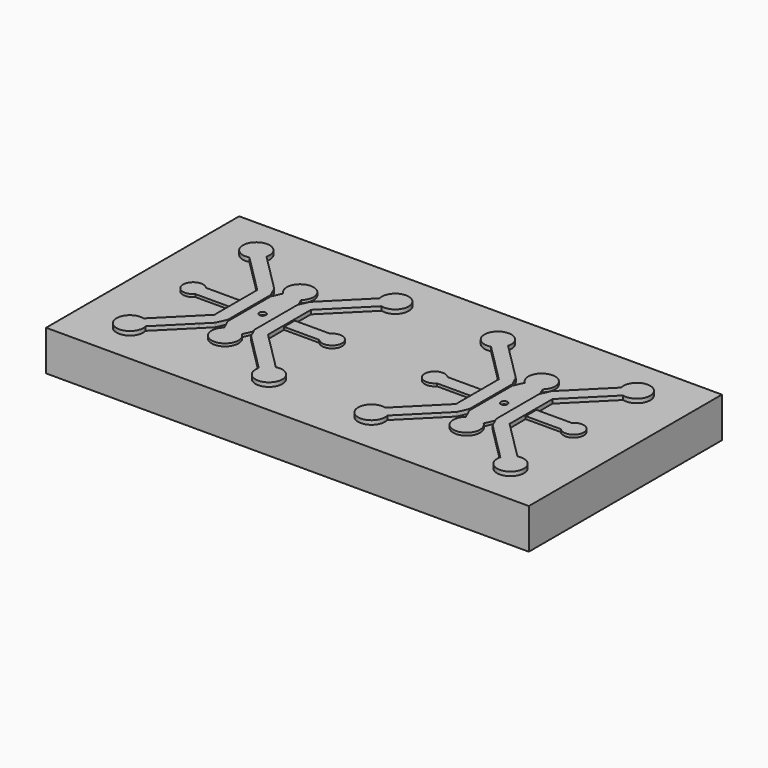
from build123d import *

# Parameters (mm, degrees)
F0_W     = 17.75
F0_H     = 18
F0_W_2   = 0.25
F1_DEPTH = 3
F2_DEPTH = 0.3
F3_DEPTH = 0.2


# Not quite as in the source:
# - a feature names something its author has since deleted; it is built from what else it names


with BuildPart() as f1:
    # F0 (on Top) → F1 (new body)
    with BuildSketch(Plane.XY):
        with Locations((8.875, 9)):
            Rectangle(F0_W, F0_H)
        with BuildLine():
            Line((9.6533412223, 11.6952957055), (9.9919033945, 10.9452957055))
            Line((9.9919033945, 10.9452957055), (10.3304655668, 11.6952957055))
            Line((10.3304655668, 11.6952957055), (10.9904227081, 12.3580254744))
            Line((10.9904227081, 12.3580254744), (13.2079580316, 14.5755632326))
            ThreePointArc((13.2079580316, 14.5755632326), (14.8809903029, 15.5414897832), (13.9150646707, 13.8684569817))
            Line((13.9150646707, 13.8684569817), (10.9919033945, 10.9452957055))
            Line((10.9919033945, 10.9452957055), (10.9919033945, 9.4452957055))
            Line((10.9919033945, 9.4452957055), (13.6148667214, 9.4452957055))
            ThreePointArc((13.6148667214, 9.4452957055), (13.70376764, 9.5296679116), (13.8052234095, 9.5984339593))
            ThreePointArc((13.8052234095, 9.5984339593), (14.9138690208, 8.823141097), (13.6148667214, 8.4452957055))
            Line((13.6148667214, 8.4452957055), (10.9919033945, 8.4452957055))
            Line((10.9919033945, 8.4452957055), (10.9919033945, 6.9452957055))
            Line((10.9919033945, 6.9452957055), (13.9150646707, 4.0221344294))
            ThreePointArc((13.9150646707, 4.0221344294), (14.8809903029, 2.3491016278), (13.2079580316, 3.3150281785))
            Line((13.2079580316, 3.3150281785), (10.9904227081, 5.5325659367))
            Line((10.9904227081, 5.5325659367), (10.3304655668, 6.1952957055))
            Line((10.3304655668, 6.1952957055), (9.9919033945, 6.9452957055))
            Line((9.9919033945, 6.9452957055), (9.6533412223, 6.1952957055))
            ThreePointArc((9.6533412223, 6.1952957055), (8.9919033945, 4.4452957055), (8.3304655668, 6.1952957055))
            Line((8.3304655668, 6.1952957055), (7.9919033945, 6.9452957055))
            Line((7.9919033945, 6.9452957055), (7.6533412223, 6.1952957055))
            Line((7.6533412223, 6.1952957055), (6.993384081, 5.5325659367))
            Line((6.993384081, 5.5325659367), (4.7758487575, 3.3150281785))
            ThreePointArc((4.7758487575, 3.3150281785), (3.1028164862, 2.3491016278), (4.0687421184, 4.0221344294))
            Line((4.0687421184, 4.0221344294), (6.9919033945, 6.9452957055))
            Line((6.9919033945, 6.9452957055), (6.9919033945, 8.4452957055))
            Line((6.9919033945, 8.4452957055), (4.3689400677, 8.4452957055))
            ThreePointArc((4.3689400677, 8.4452957055), (3.0699377683, 8.823141097), (4.1785833795, 9.5984339593))
            ThreePointArc((4.1785833795, 9.5984339593), (4.2800391491, 9.5296679116), (4.3689400677, 9.4452957055))
            Line((4.3689400677, 9.4452957055), (6.9919033945, 9.4452957055))
            Line((6.9919033945, 9.4452957055), (6.9919033945, 10.9452957055))
            Line((6.9919033945, 10.9452957055), (4.0687421184, 13.8684569817))
            ThreePointArc((4.0687421184, 13.8684569817), (3.1028164862, 15.5414897832), (4.7758487575, 14.5755632326))
            Line((4.7758487575, 14.5755632326), (6.993384081, 12.3580254744))
            Line((6.993384081, 12.3580254744), (7.6533412223, 11.6952957055))
            Line((7.6533412223, 11.6952957055), (7.9919033945, 10.9452957055))
            Line((7.9919033945, 10.9452957055), (8.3304655668, 11.6952957055))
            ThreePointArc((8.3304655668, 11.6952957055), (8.9919033945, 13.4452957055), (9.6533412223, 11.6952957055))
        make_face(mode=Mode.SUBTRACT)
        with Locations((27.125, 9)):
            Rectangle(F0_W, F0_H)
        with BuildLine():
            Line((27.6695344332, 11.6952957055), (28.0080966055, 10.9452957055))
            Line((28.0080966055, 10.9452957055), (28.3466587777, 11.6952957055))
            Line((28.3466587777, 11.6952957055), (29.006615919, 12.3580254744))
            Line((29.006615919, 12.3580254744), (31.2241512425, 14.5755632326))
            ThreePointArc((31.2241512425, 14.5755632326), (32.8971835138, 15.5414897832), (31.9312578816, 13.8684569817))
            Line((31.9312578816, 13.8684569817), (29.0080966055, 10.9452957055))
            Line((29.0080966055, 10.9452957055), (29.0080966055, 9.4452957055))
            Line((29.0080966055, 9.4452957055), (31.6310599323, 9.4452957055))
            ThreePointArc((31.6310599323, 9.4452957055), (31.7199608509, 9.5296679116), (31.8214166205, 9.5984339593))
            ThreePointArc((31.8214166205, 9.5984339593), (32.9300622317, 8.823141097), (31.6310599323, 8.4452957055))
            Line((31.6310599323, 8.4452957055), (29.0080966055, 8.4452957055))
            Line((29.0080966055, 8.4452957055), (29.0080966055, 6.9452957055))
            Line((29.0080966055, 6.9452957055), (31.9312578816, 4.0221344294))
            ThreePointArc((31.9312578816, 4.0221344294), (32.8971835138, 2.3491016278), (31.2241512425, 3.3150281785))
            Line((31.2241512425, 3.3150281785), (29.006615919, 5.5325659367))
            Line((29.006615919, 5.5325659367), (28.3466587777, 6.1952957055))
            Line((28.3466587777, 6.1952957055), (28.0080966055, 6.9452957055))
            Line((28.0080966055, 6.9452957055), (27.6695344332, 6.1952957055))
            ThreePointArc((27.6695344332, 6.1952957055), (27.0080966055, 4.4452957055), (26.3466587777, 6.1952957055))
            Line((26.3466587777, 6.1952957055), (26.0080966055, 6.9452957055))
            Line((26.0080966055, 6.9452957055), (25.6695344332, 6.1952957055))
            Line((25.6695344332, 6.1952957055), (25.0095772919, 5.5325659367))
            Line((25.0095772919, 5.5325659367), (22.7920419684, 3.3150281785))
            ThreePointArc((22.7920419684, 3.3150281785), (21.1190096971, 2.3491016278), (22.0849353293, 4.0221344294))
            Line((22.0849353293, 4.0221344294), (25.0080966055, 6.9452957055))
            Line((25.0080966055, 6.9452957055), (25.0080966055, 8.4452957055))
            Line((25.0080966055, 8.4452957055), (22.3851332786, 8.4452957055))
            ThreePointArc((22.3851332786, 8.4452957055), (21.0861309792, 8.823141097), (22.1947765905, 9.5984339593))
            ThreePointArc((22.1947765905, 9.5984339593), (22.29623236, 9.5296679116), (22.3851332786, 9.4452957055))
            Line((22.3851332786, 9.4452957055), (25.0080966055, 9.4452957055))
            Line((25.0080966055, 9.4452957055), (25.0080966055, 10.9452957055))
            Line((25.0080966055, 10.9452957055), (22.0849353293, 13.8684569817))
            ThreePointArc((22.0849353293, 13.8684569817), (21.1190096971, 15.5414897832), (22.7920419684, 14.5755632326))
            Line((22.7920419684, 14.5755632326), (25.0095772919, 12.3580254744))
            Line((25.0095772919, 12.3580254744), (25.6695344332, 11.6952957055))
            Line((25.6695344332, 11.6952957055), (26.0080966055, 10.9452957055))
            Line((26.0080966055, 10.9452957055), (26.3466587777, 11.6952957055))
            ThreePointArc((26.3466587777, 11.6952957055), (27.0080966055, 13.4452957055), (27.6695344332, 11.6952957055))
        make_face(mode=Mode.SUBTRACT)
        with BuildLine():
            Line((26.0080966055, 8.9452957055), (26.0080966055, 10.9452957055))
            Line((26.0080966055, 10.9452957055), (25.6695344332, 11.6952957055))
            Line((25.6695344332, 11.6952957055), (25.0095772919, 12.3580254744))
            Line((25.0095772919, 12.3580254744), (22.7920419684, 14.5755632326))
            ThreePointArc((22.7920419684, 14.5755632326), (21.1190096971, 15.5414897832), (22.0849353293, 13.8684569817))
            Line((22.0849353293, 13.8684569817), (25.0080966055, 10.9452957055))
            Line((25.0080966055, 10.9452957055), (25.0080966055, 9.4452957055))
            Line((25.0080966055, 9.4452957055), (25.0080966055, 8.9452957055))
            Line((25.0080966055, 8.9452957055), (25.0080966055, 8.4452957055))
            Line((25.0080966055, 8.4452957055), (25.0080966055, 6.9452957055))
            Line((25.0080966055, 6.9452957055), (22.0849353293, 4.0221344294))
            ThreePointArc((22.0849353293, 4.0221344294), (21.1190096971, 2.3491016278), (22.7920419684, 3.3150281785))
            Line((22.7920419684, 3.3150281785), (25.0095772919, 5.5325659367))
            Line((25.0095772919, 5.5325659367), (25.6695344332, 6.1952957055))
            Line((25.6695344332, 6.1952957055), (26.0080966055, 6.9452957055))
            Line((26.0080966055, 6.9452957055), (26.0080966055, 8.9452957055))
        make_face()
        with BuildLine():
            Line((28.3466587777, 11.6952957055), (28.0080966055, 10.9452957055))
            Line((28.0080966055, 10.9452957055), (28.0080966055, 8.9452957055))
            Line((28.0080966055, 8.9452957055), (28.0080966055, 6.9452957055))
            Line((28.0080966055, 6.9452957055), (28.3466587777, 6.1952957055))
            Line((28.3466587777, 6.1952957055), (29.006615919, 5.5325659367))
            Line((29.006615919, 5.5325659367), (31.2241512425, 3.3150281785))
            ThreePointArc((31.2241512425, 3.3150281785), (32.8971835138, 2.3491016278), (31.9312578816, 4.0221344294))
            Line((31.9312578816, 4.0221344294), (29.0080966055, 6.9452957055))
            Line((29.0080966055, 6.9452957055), (29.0080966055, 8.4452957055))
            Line((29.0080966055, 8.4452957055), (29.0080966055, 8.9452957055))
            Line((29.0080966055, 8.9452957055), (29.0080966055, 9.4452957055))
            Line((29.0080966055, 9.4452957055), (29.0080966055, 10.9452957055))
            Line((29.0080966055, 10.9452957055), (31.9312578816, 13.8684569817))
            ThreePointArc((31.9312578816, 13.8684569817), (32.8971835138, 15.5414897832), (31.2241512425, 14.5755632326))
            Line((31.2241512425, 14.5755632326), (29.006615919, 12.3580254744))
            Line((29.006615919, 12.3580254744), (28.3466587777, 11.6952957055))
        make_face()
        with BuildLine():
            Line((7.9919033945, 8.9452957055), (7.9919033945, 10.9452957055))
            Line((7.9919033945, 10.9452957055), (7.6533412223, 11.6952957055))
            Line((7.6533412223, 11.6952957055), (6.993384081, 12.3580254744))
            Line((6.993384081, 12.3580254744), (4.7758487575, 14.5755632326))
            ThreePointArc((4.7758487575, 14.5755632326), (3.1028164862, 15.5414897832), (4.0687421184, 13.8684569817))
            Line((4.0687421184, 13.8684569817), (6.9919033945, 10.9452957055))
            Line((6.9919033945, 10.9452957055), (6.9919033945, 9.4452957055))
            Line((6.9919033945, 9.4452957055), (6.9919033945, 8.9452957055))
            Line((6.9919033945, 8.9452957055), (6.9919033945, 8.4452957055))
            Line((6.9919033945, 8.4452957055), (6.9919033945, 6.9452957055))
            Line((6.9919033945, 6.9452957055), (4.0687421184, 4.0221344294))
            ThreePointArc((4.0687421184, 4.0221344294), (3.1028164862, 2.3491016278), (4.7758487575, 3.3150281785))
            Line((4.7758487575, 3.3150281785), (6.993384081, 5.5325659367))
            Line((6.993384081, 5.5325659367), (7.6533412223, 6.1952957055))
            Line((7.6533412223, 6.1952957055), (7.9919033945, 6.9452957055))
            Line((7.9919033945, 6.9452957055), (7.9919033945, 8.9452957055))
        make_face()
        with BuildLine():
            Line((9.9919033945, 10.9452957055), (9.9919033945, 8.9452957055))
            Line((9.9919033945, 8.9452957055), (9.9919033945, 6.9452957055))
            Line((9.9919033945, 6.9452957055), (10.3304655668, 6.1952957055))
            Line((10.3304655668, 6.1952957055), (10.9904227081, 5.5325659367))
            Line((10.9904227081, 5.5325659367), (13.2079580316, 3.3150281785))
            ThreePointArc((13.2079580316, 3.3150281785), (14.8809903029, 2.3491016278), (13.9150646707, 4.0221344294))
            Line((13.9150646707, 4.0221344294), (10.9919033945, 6.9452957055))
            Line((10.9919033945, 6.9452957055), (10.9919033945, 8.4452957055))
            Line((10.9919033945, 8.4452957055), (10.9919033945, 8.9452957055))
            Line((10.9919033945, 8.9452957055), (10.9919033945, 9.4452957055))
            Line((10.9919033945, 9.4452957055), (10.9919033945, 10.9452957055))
            Line((10.9919033945, 10.9452957055), (13.9150646707, 13.8684569817))
            ThreePointArc((13.9150646707, 13.8684569817), (14.8809903029, 15.5414897832), (13.2079580316, 14.5755632326))
            Line((13.2079580316, 14.5755632326), (10.9904227081, 12.3580254744))
            Line((10.9904227081, 12.3580254744), (10.3304655668, 11.6952957055))
            Line((10.3304655668, 11.6952957055), (9.9919033945, 10.9452957055))
        make_face()
        with BuildLine():
            Line((28.0080966055, 8.9452957055), (28.0080966055, 10.9452957055))
            Line((28.0080966055, 10.9452957055), (27.6695344332, 11.6952957055))
            ThreePointArc((27.6695344332, 11.6952957055), (27.0080966055, 13.4452957055), (26.3466587777, 11.6952957055))
            Line((26.3466587777, 11.6952957055), (26.0080966055, 10.9452957055))
            Line((26.0080966055, 10.9452957055), (26.0080966055, 8.9452957055))
            Line((26.0080966055, 8.9452957055), (26.0080966055, 6.9452957055))
            Line((26.0080966055, 6.9452957055), (26.3466587777, 6.1952957055))
            ThreePointArc((26.3466587777, 6.1952957055), (27.0080966055, 4.4452957055), (27.6695344332, 6.1952957055))
            Line((27.6695344332, 6.1952957055), (28.0080966055, 6.9452957055))
            Line((28.0080966055, 6.9452957055), (28.0080966055, 8.9452957055))
        make_face()
        with BuildLine():
            ThreePointArc((27.0080966055, 9.1952957055), (27.1848733008, 9.1220724008), (27.2580966055, 8.9452957055))
            ThreePointArc((27.2580966055, 8.9452957055), (27.1848733008, 8.7685190102), (27.0080966055, 8.6952957055))
            ThreePointArc((27.0080966055, 8.6952957055), (26.7580966055, 8.9452957055), (27.0080966055, 9.1952957055))
        make_face(mode=Mode.SUBTRACT)
        with BuildLine():
            Line((9.9919033945, 6.9452957055), (9.9919033945, 8.9452957055))
            Line((9.9919033945, 8.9452957055), (9.9919033945, 10.9452957055))
            Line((9.9919033945, 10.9452957055), (9.6533412223, 11.6952957055))
            ThreePointArc((9.6533412223, 11.6952957055), (8.9919033945, 13.4452957055), (8.3304655668, 11.6952957055))
            Line((8.3304655668, 11.6952957055), (7.9919033945, 10.9452957055))
            Line((7.9919033945, 10.9452957055), (7.9919033945, 8.9452957055))
            Line((7.9919033945, 8.9452957055), (7.9919033945, 6.9452957055))
            Line((7.9919033945, 6.9452957055), (8.3304655668, 6.1952957055))
            ThreePointArc((8.3304655668, 6.1952957055), (8.9919033945, 4.4452957055), (9.6533412223, 6.1952957055))
            Line((9.6533412223, 6.1952957055), (9.9919033945, 6.9452957055))
        make_face()
        with BuildLine():
            ThreePointArc((8.9919033945, 9.1952957055), (9.1686800898, 9.1220724008), (9.2419033945, 8.9452957055))
            ThreePointArc((9.2419033945, 8.9452957055), (9.1686800898, 8.7685190102), (8.9919033945, 8.6952957055))
            ThreePointArc((8.9919033945, 8.6952957055), (8.7419033945, 8.9452957055), (8.9919033945, 9.1952957055))
        make_face(mode=Mode.SUBTRACT)
        with Locations((17.875, 9)):
            Rectangle(F0_W_2, F0_H)
        with Locations((18.125, 9)):
            Rectangle(F0_W_2, F0_H)
        with BuildLine():
            Line((6.9919033945, 8.9452957055), (6.9919033945, 9.4452957055))
            Line((6.9919033945, 9.4452957055), (4.3689400677, 9.4452957055))
            ThreePointArc((4.3689400677, 9.4452957055), (4.2800391491, 9.5296679116), (4.1785833795, 9.5984339593))
            ThreePointArc((4.1785833795, 9.5984339593), (3.0699377683, 8.823141097), (4.3689400677, 8.4452957055))
            Line((4.3689400677, 8.4452957055), (6.9919033945, 8.4452957055))
            Line((6.9919033945, 8.4452957055), (6.9919033945, 8.9452957055))
        make_face()
        with BuildLine():
            Line((31.6310599323, 9.4452957055), (29.0080966055, 9.4452957055))
            Line((29.0080966055, 9.4452957055), (29.0080966055, 8.9452957055))
            Line((29.0080966055, 8.9452957055), (29.0080966055, 8.4452957055))
            Line((29.0080966055, 8.4452957055), (31.6310599323, 8.4452957055))
            ThreePointArc((31.6310599323, 8.4452957055), (32.9300622317, 8.823141097), (31.8214166205, 9.5984339593))
            ThreePointArc((31.8214166205, 9.5984339593), (31.7199608509, 9.5296679116), (31.6310599323, 9.4452957055))
        make_face()
        with BuildLine():
            Line((25.0080966055, 8.9452957055), (25.0080966055, 9.4452957055))
            Line((25.0080966055, 9.4452957055), (22.3851332786, 9.4452957055))
            ThreePointArc((22.3851332786, 9.4452957055), (22.29623236, 9.5296679116), (22.1947765905, 9.5984339593))
            ThreePointArc((22.1947765905, 9.5984339593), (21.0861309792, 8.823141097), (22.3851332786, 8.4452957055))
            Line((22.3851332786, 8.4452957055), (25.0080966055, 8.4452957055))
            Line((25.0080966055, 8.4452957055), (25.0080966055, 8.9452957055))
        make_face()
        with BuildLine():
            Line((13.6148667214, 9.4452957055), (10.9919033945, 9.4452957055))
            Line((10.9919033945, 9.4452957055), (10.9919033945, 8.9452957055))
            Line((10.9919033945, 8.9452957055), (10.9919033945, 8.4452957055))
            Line((10.9919033945, 8.4452957055), (13.6148667214, 8.4452957055))
            ThreePointArc((13.6148667214, 8.4452957055), (14.9138690208, 8.823141097), (13.8052234095, 9.5984339593))
            ThreePointArc((13.8052234095, 9.5984339593), (13.70376764, 9.5296679116), (13.6148667214, 9.4452957055))
        make_face()
        with BuildLine():
            ThreePointArc((8.9919033945, 8.6952957055), (9.1686800898, 8.7685190102), (9.2419033945, 8.9452957055))
            ThreePointArc((9.2419033945, 8.9452957055), (9.1686800898, 9.1220724008), (8.9919033945, 9.1952957055))
            Line((8.9919033945, 9.1952957055), (8.9919033945, 8.6952957055))
        make_face()
        with BuildLine():
            ThreePointArc((27.0080966055, 8.6952957055), (27.1848733008, 8.7685190102), (27.2580966055, 8.9452957055))
            ThreePointArc((27.2580966055, 8.9452957055), (27.1848733008, 9.1220724008), (27.0080966055, 9.1952957055))
            Line((27.0080966055, 9.1952957055), (27.0080966055, 8.6952957055))
        make_face()
        with BuildLine():
            Line((8.9919033945, 8.6952957055), (8.9919033945, 9.1952957055))
            ThreePointArc((8.9919033945, 9.1952957055), (8.7419033945, 8.9452957055), (8.9919033945, 8.6952957055))
        make_face()
        with BuildLine():
            Line((27.0080966055, 8.6952957055), (27.0080966055, 9.1952957055))
            ThreePointArc((27.0080966055, 9.1952957055), (26.7580966055, 8.9452957055), (27.0080966055, 8.6952957055))
        make_face()
    extrude(amount=-F1_DEPTH)

    # F0 (on Top) → F2 (join)
    with BuildSketch(Plane.XY):
        with BuildLine():
            Line((7.9919033945, 8.9452957055), (7.9919033945, 10.9452957055))
            Line((7.9919033945, 10.9452957055), (7.6533412223, 11.6952957055))
            Line((7.6533412223, 11.6952957055), (6.993384081, 12.3580254744))
            Line((6.993384081, 12.3580254744), (4.7758487575, 14.5755632326))
            ThreePointArc((4.7758487575, 14.5755632326), (3.1028164862, 15.5414897832), (4.0687421184, 13.8684569817))
            Line((4.0687421184, 13.8684569817), (6.9919033945, 10.9452957055))
            Line((6.9919033945, 10.9452957055), (6.9919033945, 9.4452957055))
            Line((6.9919033945, 9.4452957055), (6.9919033945, 8.9452957055))
            Line((6.9919033945, 8.9452957055), (6.9919033945, 8.4452957055))
            Line((6.9919033945, 8.4452957055), (6.9919033945, 6.9452957055))
            Line((6.9919033945, 6.9452957055), (4.0687421184, 4.0221344294))
            ThreePointArc((4.0687421184, 4.0221344294), (3.1028164862, 2.3491016278), (4.7758487575, 3.3150281785))
            Line((4.7758487575, 3.3150281785), (6.993384081, 5.5325659367))
            Line((6.993384081, 5.5325659367), (7.6533412223, 6.1952957055))
            Line((7.6533412223, 6.1952957055), (7.9919033945, 6.9452957055))
            Line((7.9919033945, 6.9452957055), (7.9919033945, 8.9452957055))
        make_face()
        with BuildLine():
            Line((9.9919033945, 10.9452957055), (9.9919033945, 8.9452957055))
            Line((9.9919033945, 8.9452957055), (9.9919033945, 6.9452957055))
            Line((9.9919033945, 6.9452957055), (10.3304655668, 6.1952957055))
            Line((10.3304655668, 6.1952957055), (10.9904227081, 5.5325659367))
            Line((10.9904227081, 5.5325659367), (13.2079580316, 3.3150281785))
            ThreePointArc((13.2079580316, 3.3150281785), (14.8809903029, 2.3491016278), (13.9150646707, 4.0221344294))
            Line((13.9150646707, 4.0221344294), (10.9919033945, 6.9452957055))
            Line((10.9919033945, 6.9452957055), (10.9919033945, 8.4452957055))
            Line((10.9919033945, 8.4452957055), (10.9919033945, 8.9452957055))
            Line((10.9919033945, 8.9452957055), (10.9919033945, 9.4452957055))
            Line((10.9919033945, 9.4452957055), (10.9919033945, 10.9452957055))
            Line((10.9919033945, 10.9452957055), (13.9150646707, 13.8684569817))
            ThreePointArc((13.9150646707, 13.8684569817), (14.8809903029, 15.5414897832), (13.2079580316, 14.5755632326))
            Line((13.2079580316, 14.5755632326), (10.9904227081, 12.3580254744))
            Line((10.9904227081, 12.3580254744), (10.3304655668, 11.6952957055))
            Line((10.3304655668, 11.6952957055), (9.9919033945, 10.9452957055))
        make_face()
        with BuildLine():
            Line((26.0080966055, 8.9452957055), (26.0080966055, 10.9452957055))
            Line((26.0080966055, 10.9452957055), (25.6695344332, 11.6952957055))
            Line((25.6695344332, 11.6952957055), (25.0095772919, 12.3580254744))
            Line((25.0095772919, 12.3580254744), (22.7920419684, 14.5755632326))
            ThreePointArc((22.7920419684, 14.5755632326), (21.1190096971, 15.5414897832), (22.0849353293, 13.8684569817))
            Line((22.0849353293, 13.8684569817), (25.0080966055, 10.9452957055))
            Line((25.0080966055, 10.9452957055), (25.0080966055, 9.4452957055))
            Line((25.0080966055, 9.4452957055), (25.0080966055, 8.9452957055))
            Line((25.0080966055, 8.9452957055), (25.0080966055, 8.4452957055))
            Line((25.0080966055, 8.4452957055), (25.0080966055, 6.9452957055))
            Line((25.0080966055, 6.9452957055), (22.0849353293, 4.0221344294))
            ThreePointArc((22.0849353293, 4.0221344294), (21.1190096971, 2.3491016278), (22.7920419684, 3.3150281785))
            Line((22.7920419684, 3.3150281785), (25.0095772919, 5.5325659367))
            Line((25.0095772919, 5.5325659367), (25.6695344332, 6.1952957055))
            Line((25.6695344332, 6.1952957055), (26.0080966055, 6.9452957055))
            Line((26.0080966055, 6.9452957055), (26.0080966055, 8.9452957055))
        make_face()
        with BuildLine():
            Line((28.3466587777, 11.6952957055), (28.0080966055, 10.9452957055))
            Line((28.0080966055, 10.9452957055), (28.0080966055, 8.9452957055))
            Line((28.0080966055, 8.9452957055), (28.0080966055, 6.9452957055))
            Line((28.0080966055, 6.9452957055), (28.3466587777, 6.1952957055))
            Line((28.3466587777, 6.1952957055), (29.006615919, 5.5325659367))
            Line((29.006615919, 5.5325659367), (31.2241512425, 3.3150281785))
            ThreePointArc((31.2241512425, 3.3150281785), (32.8971835138, 2.3491016278), (31.9312578816, 4.0221344294))
            Line((31.9312578816, 4.0221344294), (29.0080966055, 6.9452957055))
            Line((29.0080966055, 6.9452957055), (29.0080966055, 8.4452957055))
            Line((29.0080966055, 8.4452957055), (29.0080966055, 8.9452957055))
            Line((29.0080966055, 8.9452957055), (29.0080966055, 9.4452957055))
            Line((29.0080966055, 9.4452957055), (29.0080966055, 10.9452957055))
            Line((29.0080966055, 10.9452957055), (31.9312578816, 13.8684569817))
            ThreePointArc((31.9312578816, 13.8684569817), (32.8971835138, 15.5414897832), (31.2241512425, 14.5755632326))
            Line((31.2241512425, 14.5755632326), (29.006615919, 12.3580254744))
            Line((29.006615919, 12.3580254744), (28.3466587777, 11.6952957055))
        make_face()
    extrude(amount=F2_DEPTH)

    # F0 (on Top) → F3 (join)
    with BuildSketch(Plane.XY):
        with BuildLine():
            Line((9.9919033945, 6.9452957055), (9.9919033945, 8.9452957055))
            Line((9.9919033945, 8.9452957055), (9.9919033945, 10.9452957055))
            Line((9.9919033945, 10.9452957055), (9.6533412223, 11.6952957055))
            ThreePointArc((9.6533412223, 11.6952957055), (8.9919033945, 13.4452957055), (8.3304655668, 11.6952957055))
            Line((8.3304655668, 11.6952957055), (7.9919033945, 10.9452957055))
            Line((7.9919033945, 10.9452957055), (7.9919033945, 8.9452957055))
            Line((7.9919033945, 8.9452957055), (7.9919033945, 6.9452957055))
            Line((7.9919033945, 6.9452957055), (8.3304655668, 6.1952957055))
            ThreePointArc((8.3304655668, 6.1952957055), (8.9919033945, 4.4452957055), (9.6533412223, 6.1952957055))
            Line((9.6533412223, 6.1952957055), (9.9919033945, 6.9452957055))
        make_face()
        with BuildLine():
            ThreePointArc((8.9919033945, 9.1952957055), (9.1686800898, 9.1220724008), (9.2419033945, 8.9452957055))
            ThreePointArc((9.2419033945, 8.9452957055), (9.1686800898, 8.7685190102), (8.9919033945, 8.6952957055))
            ThreePointArc((8.9919033945, 8.6952957055), (8.7419033945, 8.9452957055), (8.9919033945, 9.1952957055))
        make_face(mode=Mode.SUBTRACT)
        with BuildLine():
            Line((13.6148667214, 9.4452957055), (10.9919033945, 9.4452957055))
            Line((10.9919033945, 9.4452957055), (10.9919033945, 8.9452957055))
            Line((10.9919033945, 8.9452957055), (10.9919033945, 8.4452957055))
            Line((10.9919033945, 8.4452957055), (13.6148667214, 8.4452957055))
            ThreePointArc((13.6148667214, 8.4452957055), (14.9138690208, 8.823141097), (13.8052234095, 9.5984339593))
            ThreePointArc((13.8052234095, 9.5984339593), (13.70376764, 9.5296679116), (13.6148667214, 9.4452957055))
        make_face()
        with BuildLine():
            Line((6.9919033945, 8.9452957055), (6.9919033945, 9.4452957055))
            Line((6.9919033945, 9.4452957055), (4.3689400677, 9.4452957055))
            ThreePointArc((4.3689400677, 9.4452957055), (4.2800391491, 9.5296679116), (4.1785833795, 9.5984339593))
            ThreePointArc((4.1785833795, 9.5984339593), (3.0699377683, 8.823141097), (4.3689400677, 8.4452957055))
            Line((4.3689400677, 8.4452957055), (6.9919033945, 8.4452957055))
            Line((6.9919033945, 8.4452957055), (6.9919033945, 8.9452957055))
        make_face()
        with BuildLine():
            Line((25.0080966055, 8.9452957055), (25.0080966055, 9.4452957055))
            Line((25.0080966055, 9.4452957055), (22.3851332786, 9.4452957055))
            ThreePointArc((22.3851332786, 9.4452957055), (22.29623236, 9.5296679116), (22.1947765905, 9.5984339593))
            ThreePointArc((22.1947765905, 9.5984339593), (21.0861309792, 8.823141097), (22.3851332786, 8.4452957055))
            Line((22.3851332786, 8.4452957055), (25.0080966055, 8.4452957055))
            Line((25.0080966055, 8.4452957055), (25.0080966055, 8.9452957055))
        make_face()
        with BuildLine():
            Line((28.0080966055, 8.9452957055), (28.0080966055, 10.9452957055))
            Line((28.0080966055, 10.9452957055), (27.6695344332, 11.6952957055))
            ThreePointArc((27.6695344332, 11.6952957055), (27.0080966055, 13.4452957055), (26.3466587777, 11.6952957055))
            Line((26.3466587777, 11.6952957055), (26.0080966055, 10.9452957055))
            Line((26.0080966055, 10.9452957055), (26.0080966055, 8.9452957055))
            Line((26.0080966055, 8.9452957055), (26.0080966055, 6.9452957055))
            Line((26.0080966055, 6.9452957055), (26.3466587777, 6.1952957055))
            ThreePointArc((26.3466587777, 6.1952957055), (27.0080966055, 4.4452957055), (27.6695344332, 6.1952957055))
            Line((27.6695344332, 6.1952957055), (28.0080966055, 6.9452957055))
            Line((28.0080966055, 6.9452957055), (28.0080966055, 8.9452957055))
        make_face()
        with BuildLine():
            ThreePointArc((27.0080966055, 9.1952957055), (27.1848733008, 9.1220724008), (27.2580966055, 8.9452957055))
            ThreePointArc((27.2580966055, 8.9452957055), (27.1848733008, 8.7685190102), (27.0080966055, 8.6952957055))
            ThreePointArc((27.0080966055, 8.6952957055), (26.7580966055, 8.9452957055), (27.0080966055, 9.1952957055))
        make_face(mode=Mode.SUBTRACT)
        with BuildLine():
            Line((31.6310599323, 9.4452957055), (29.0080966055, 9.4452957055))
            Line((29.0080966055, 9.4452957055), (29.0080966055, 8.9452957055))
            Line((29.0080966055, 8.9452957055), (29.0080966055, 8.4452957055))
            Line((29.0080966055, 8.4452957055), (31.6310599323, 8.4452957055))
            ThreePointArc((31.6310599323, 8.4452957055), (32.9300622317, 8.823141097), (31.8214166205, 9.5984339593))
            ThreePointArc((31.8214166205, 9.5984339593), (31.7199608509, 9.5296679116), (31.6310599323, 9.4452957055))
        make_face()
    extrude(amount=F3_DEPTH)


solid = f1.part
